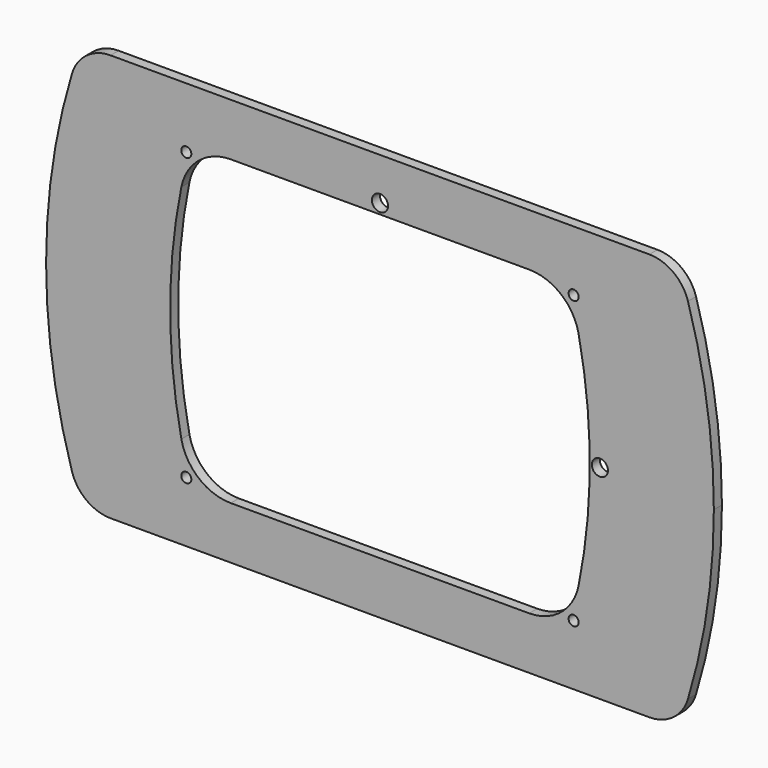
from build123d import *

# Parameters (mm, degrees)
F0_R     = 2.5
F0_R_2   = 4
F1_DEPTH = 5


# Not quite as in the source:
# - ends of sketch curves that miss each other by under 0.0002 mm in the source are joined


with BuildPart() as f1:
    # F0 (on Front) → F1 (new body)
    with BuildSketch(Plane.XZ):
        with BuildLine():
            ThreePointArc((215.3364533002, 370.0381469093), (202.5092928068, 283.2524328558), (215.3364530138, 196.4667187599))
            ThreePointArc((215.3364530138, 196.4667187599), (222.5589410473, 186.1945021744), (234.481309, 182.252433))
            Line((234.481309, 182.252433), (501.537276, 182.252433))
            ThreePointArc((501.537276, 182.252433), (513.4596440465, 186.1945022441), (520.6821320538, 196.4667189837))
            ThreePointArc((520.6821320538, 196.4667189837), (530.2851775529, 239.3881650909), (533.5092924377, 283.2524341717))
            ThreePointArc((533.5092924377, 283.2524341717), (530.2851774064, 327.11670224), (520.6821320538, 370.0381473561))
            ThreePointArc((520.6821320538, 370.0381473561), (513.4596440465, 380.3103637559), (501.537276, 384.252433))
            Line((501.537276, 384.252433), (234.481309, 384.252433))
            ThreePointArc((234.481309, 384.252433), (222.5589409535, 380.3103637559), (215.3364533002, 370.0381469093))
        make_face()
        with Locations((272.009293, 212.252433)):
            Circle(F0_R, mode=Mode.SUBTRACT)
        with BuildLine():
            ThreePointArc((466.4531644107, 228.2524329162), (457.7696552677, 213.8875162419), (441.958267, 208.252433))
            Line((441.958267, 208.252433), (294.060318, 208.252433))
            ThreePointArc((294.060318, 208.252433), (278.2489297323, 213.8875162419), (269.5654205893, 228.2524329162))
            ThreePointArc((269.5654205893, 228.2524329162), (264.009293, 283.252433), (269.5654212821, 338.2524329424))
            ThreePointArc((269.5654212821, 338.2524329424), (278.2489297323, 352.6173497581), (294.060318, 358.252433))
            Line((294.060318, 358.252433), (441.958267, 358.252433))
            ThreePointArc((441.958267, 358.252433), (457.7696552677, 352.6173497581), (466.4531644107, 338.2524330838))
            ThreePointArc((466.4531644107, 338.2524330838), (472.009293, 283.252433), (466.4531644107, 228.2524329162))
        make_face(mode=Mode.SUBTRACT)
        with Locations((272.009293, 354.252433)):
            Circle(F0_R, mode=Mode.SUBTRACT)
        with Locations((368.009293, 363.252433)):
            Circle(F0_R_2, mode=Mode.SUBTRACT)
        with Locations((464.009293, 212.252433)):
            Circle(F0_R, mode=Mode.SUBTRACT)
        with Locations((477.009293, 283.252433)):
            Circle(F0_R_2, mode=Mode.SUBTRACT)
        with Locations((464.009293, 354.252433)):
            Circle(F0_R, mode=Mode.SUBTRACT)
    extrude(amount=F1_DEPTH)


solid = f1.part
